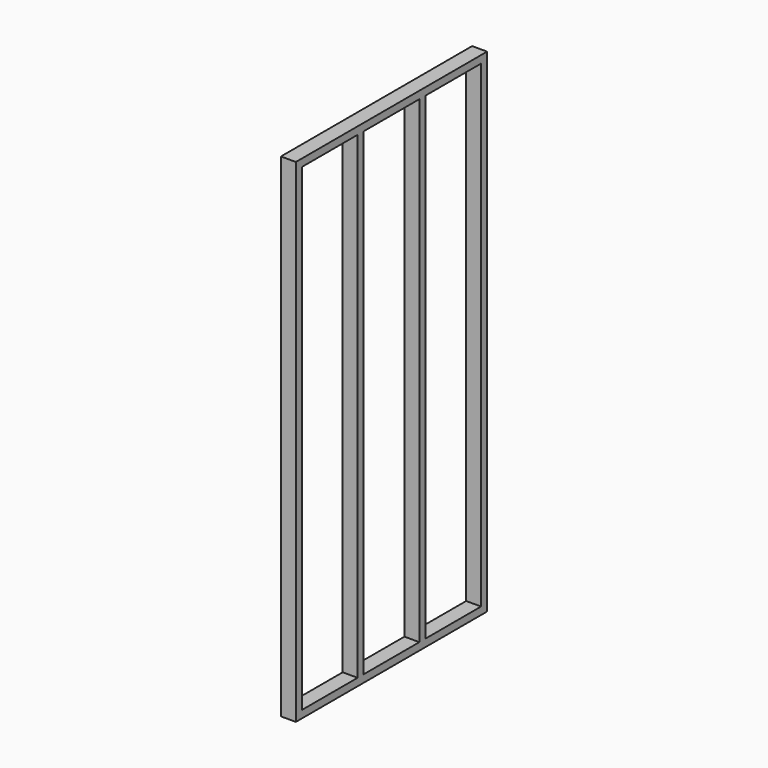
from build123d import *

# Parameters (mm, degrees)
F0_W     = 76.2
F0_H     = 1219.2
F1_DEPTH = 38.1
F2_W     = 76.2
F2_H     = 38.1
F3_DEPTH = 2438.4
F4_START = 2476.5
F4_DEPTH = 38.1


with BuildPart() as f1:
    # F0 (on Top) → F1 (new body)
    with BuildSketch(Plane.XY):
        with Locations((-79.2764335848, -16.3942715153)):
            Rectangle(F0_W, F0_H)
    extrude(amount=F1_DEPTH)

    # F2 (on face) → F3 (join)
    with BuildSketch(Plane.XY.offset(38.1)):
        with Locations((-79.2764335848, -606.9442715153)):
            Rectangle(F2_W, F2_H)
        with Locations((-79.2764335848, 574.1557284847)):
            Rectangle(F2_W, F2_H)
        with Locations((-79.2764335848, 180.4557284847)):
            Rectangle(F2_W, F2_H)
        with Locations((-79.2764335848, -213.2442715153)):
            Rectangle(F2_W, F2_H)
    extrude(amount=F3_DEPTH)

    # F0 (on Top) → F4 (join)
    with BuildSketch(Plane.XY.offset(F4_START)):
        with Locations((-79.2764335848, -16.3942715153)):
            Rectangle(F0_W, F0_H)
    extrude(amount=F4_DEPTH)


solid = f1.part
